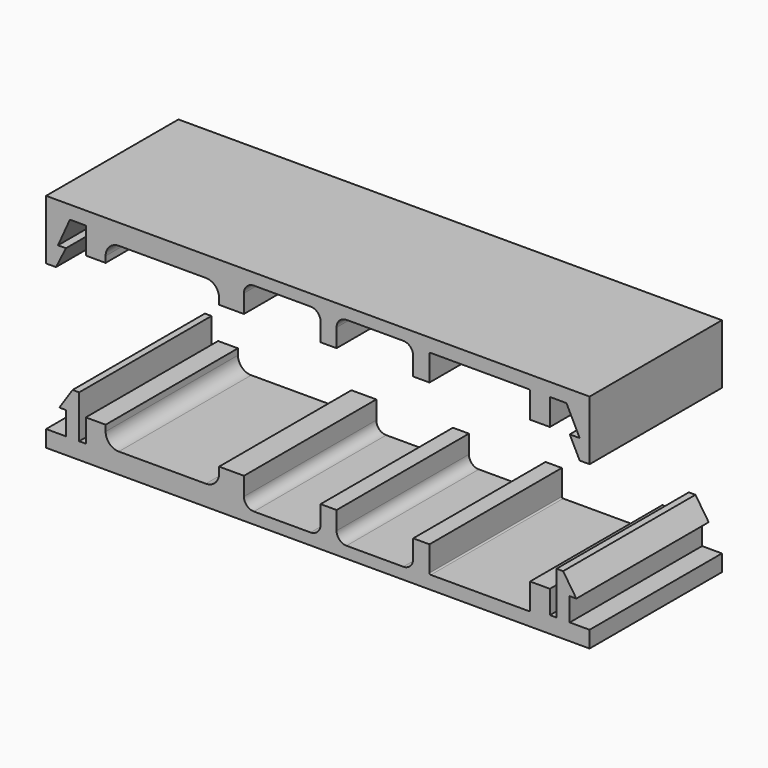
from build123d import *

# Parameters (mm, degrees)
F1_DEPTH = 25
F0_W     = 2
F0_H     = 2.5
F0_H_2   = 3.5
F2_DEPTH = 25


with BuildPart() as f1:
    # F0 (on Front) → F1 (new body)
    with BuildSketch(Plane.XZ):
        Polygon((-41.0725, 6), (-41.0725, 0), (-39.2735674977, 0), (-37.4728558326, 4), (-36.5725, 6), align=None)
        Polygon((-37.4728558326, 4), (-35.0725, 4), (-35.0725, 4.5), (-35.0725, 6), (-36.5725, 6), align=None)
        with BuildLine():
            Line((32.0725, 0), (35.0725, 0))
            Line((35.0725, 0), (35.0725, 4))
            Line((35.0725, 4), (35.0725, 4.5))
            Line((35.0725, 4.5), (35.0725, 6))
            Line((35.0725, 6), (33.5725, 6))
            Line((33.5725, 6), (-33.5725, 6))
            Line((-33.5725, 6), (-35.0725, 6))
            Line((-35.0725, 6), (-35.0725, 4.5))
            Line((-35.0725, 4.5), (-35.0725, 4))
            Line((-35.0725, 4), (-35.0725, 0))
            Line((-35.0725, 0), (-32.0725, 0))
            Line((-32.0725, 0), (-32.0725, 0.925))
            ThreePointArc((-32.0725, 0.925), (-31.4867135624, 2.3392135624), (-30.0725, 2.925))
            Line((-30.0725, 2.925), (-16.9225, 2.925))
            ThreePointArc((-16.9225, 2.925), (-15.5082864376, 2.3392135624), (-14.9225, 0.925))
            Line((-14.9225, 0.925), (-14.9225, 0))
            Line((-14.9225, 0), (-11.1675, 0))
            Line((-11.1675, 0), (-11.1675, 2.765))
            ThreePointArc((-11.1675, 2.765), (-10.7281601718, 3.8256601718), (-9.6675, 4.265))
            Line((-9.6675, 4.265), (-1.0875, 4.265))
            ThreePointArc((-1.0875, 4.265), (-0.0268398282, 3.8256601718), (0.4125, 2.765))
            Line((0.4125, 2.765), (0.4125, 0))
            Line((0.4125, 0), (2.8325, 0))
            Line((2.8325, 0), (2.8325, 2.765))
            ThreePointArc((2.8325, 2.765), (3.2718398282, 3.8256601718), (4.3325, 4.265))
            Line((4.3325, 4.265), (12.9125, 4.265))
            ThreePointArc((12.9125, 4.265), (13.9731601718, 3.8256601718), (14.4125, 2.765))
            Line((14.4125, 2.765), (14.4125, 0))
            Line((14.4125, 0), (16.8725, 0))
            Line((16.8725, 0), (16.8725, 3.8))
            ThreePointArc((16.8725, 3.8), (16.9310786438, 3.9414213562), (17.0725, 4))
            Line((17.0725, 4), (31.8725, 4))
            ThreePointArc((31.8725, 4), (32.0139213562, 3.9414213562), (32.0725, 3.8))
            Line((32.0725, 3.8), (32.0725, 0))
        make_face()
        Polygon((35.0725, 4.5), (35.0725, 4), (37.5725, 4), (36.5725, 6), (35.0725, 6), align=None)
        Polygon((39.5725, 0), (41.0725, 0), (41.0725, 6), (36.5725, 6), (37.5725, 4), align=None)
        Polygon((39.5725, -3), (41.0725, -3), (41.0725, 0), (39.5725, 0), (38.0725, 0), align=None)
        Polygon((-41.0725, 0), (-41.0725, -3), (-39.5725, -3), (-38.0725, 0), (-39.2735674977, 0), align=None)
    extrude(amount=F1_DEPTH)


with BuildPart() as f2:
    # F0 (on Front) → F2 (new body)
    with BuildSketch(Plane.XZ):
        with BuildLine():
            Line((-33.572499007, -27.5272362262), (33.572500993, -27.5272362262))
            Line((33.572500993, -27.5272362262), (35.072500993, -27.5272362262))
            Line((35.072500993, -27.5272362262), (35.072500993, -26.0272362262))
            Line((35.072500993, -26.0272362262), (35.072500993, -25.0272362262))
            Line((35.072500993, -25.0272362262), (35.072500993, -21.5272362262))
            Line((35.072500993, -21.5272362262), (32.072500993, -21.5272362262))
            Line((32.072500993, -21.5272362262), (32.072500993, -25.3272362262))
            ThreePointArc((32.072500993, -25.3272362262), (32.0139223493, -25.4686575824), (31.872500993, -25.5272362262))
            Line((31.872500993, -25.5272362262), (17.072500993, -25.5272362262))
            ThreePointArc((17.072500993, -25.5272362262), (16.9310796368, -25.4686575824), (16.872500993, -25.3272362262))
            Line((16.872500993, -25.3272362262), (16.872500993, -21.5272362262))
            Line((16.872500993, -21.5272362262), (14.412500993, -21.5272362262))
            Line((14.412500993, -21.5272362262), (14.412500993, -24.2922362262))
            ThreePointArc((14.412500993, -24.2922362262), (13.9731611648, -25.352896398), (12.912500993, -25.7922362262))
            Line((12.912500993, -25.7922362262), (4.332500993, -25.7922362262))
            ThreePointArc((4.332500993, -25.7922362262), (3.2718408212, -25.352896398), (2.832500993, -24.2922362262))
            Line((2.832500993, -24.2922362262), (2.832500993, -21.5272362262))
            Line((2.832500993, -21.5272362262), (0.412500993, -21.5272362262))
            Line((0.412500993, -21.5272362262), (0.412500993, -24.2922362262))
            ThreePointArc((0.412500993, -24.2922362262), (-0.0268388352, -25.352896398), (-1.087499007, -25.7922362262))
            Line((-1.087499007, -25.7922362262), (-9.667499007, -25.7922362262))
            ThreePointArc((-9.667499007, -25.7922362262), (-10.7281591788, -25.352896398), (-11.167499007, -24.2922362262))
            Line((-11.167499007, -24.2922362262), (-11.167499007, -21.5272362262))
            Line((-11.167499007, -21.5272362262), (-14.922499007, -21.5272362262))
            Line((-14.922499007, -21.5272362262), (-14.922499007, -22.4522362262))
            ThreePointArc((-14.922499007, -22.4522362262), (-15.5082854446, -23.8664497886), (-16.922499007, -24.4522362262))
            Line((-16.922499007, -24.4522362262), (-30.072499007, -24.4522362262))
            ThreePointArc((-30.072499007, -24.4522362262), (-31.4867125694, -23.8664497886), (-32.072499007, -22.4522362262))
            Line((-32.072499007, -22.4522362262), (-32.072499007, -21.5272362262))
            Line((-32.072499007, -21.5272362262), (-35.072499007, -21.5272362262))
            Line((-35.072499007, -21.5272362262), (-35.072499007, -25.0272362262))
            Line((-35.072499007, -25.0272362262), (-35.072499007, -26.0272362262))
            Line((-35.072499007, -26.0272362262), (-35.072499007, -27.5272362262))
            Line((-35.072499007, -27.5272362262), (-33.572499007, -27.5272362262))
        make_face()
        Polygon((35.072500993, -26.0272362262), (35.072500993, -27.5272362262), (36.072500993, -27.5272362262), (36.072500993, -25.0272362262), (35.072500993, -25.0272362262), align=None)
        Polygon((-36.072499007, -27.5272362262), (-35.072499007, -27.5272362262), (-35.072499007, -26.0272362262), (-35.072499007, -25.0272362262), (-36.072499007, -25.0272362262), align=None)
        with Locations((37.072500993, -26.2772362262)):
            Rectangle(F0_W, F0_H)
        with Locations((-37.072499007, -26.2772362262)):
            Rectangle(F0_W, F0_H)
        Polygon((38.072500993, -25.0272362262), (38.072500993, -27.5272362262), (41.072500993, -27.5272362262), (39.822500993, -25.0272362262), align=None)
        with Locations((37.072500993, -23.2772362262)):
            Rectangle(F0_W, F0_H_2)
        Polygon((-41.072499007, -27.5272362262), (-38.072499007, -27.5272362262), (-38.072499007, -25.0272362262), (-39.822499007, -25.0272362262), align=None)
        with Locations((-37.072499007, -23.2772362262)):
            Rectangle(F0_W, F0_H_2)
        Polygon((39.822500993, -25.0272362262), (41.072500993, -27.5272362262), (41.072500993, -25.0272362262), align=None)
        Polygon((36.072500993, -18.5272362262), (36.072500993, -21.5272362262), (38.072500993, -21.5272362262), (39.072500993, -21.5272362262), (37.072500993, -18.5272362262), align=None)
        Polygon((-41.072499007, -25.0272362262), (-41.072499007, -27.5272362262), (-39.822499007, -25.0272362262), align=None)
        Polygon((-38.072499007, -21.5272362262), (-36.072499007, -21.5272362262), (-36.072499007, -18.5272362262), (-37.072499007, -18.5272362262), (-39.072499007, -21.5272362262), align=None)
    extrude(amount=F2_DEPTH)


solid = Compound([f1.part, f2.part])
